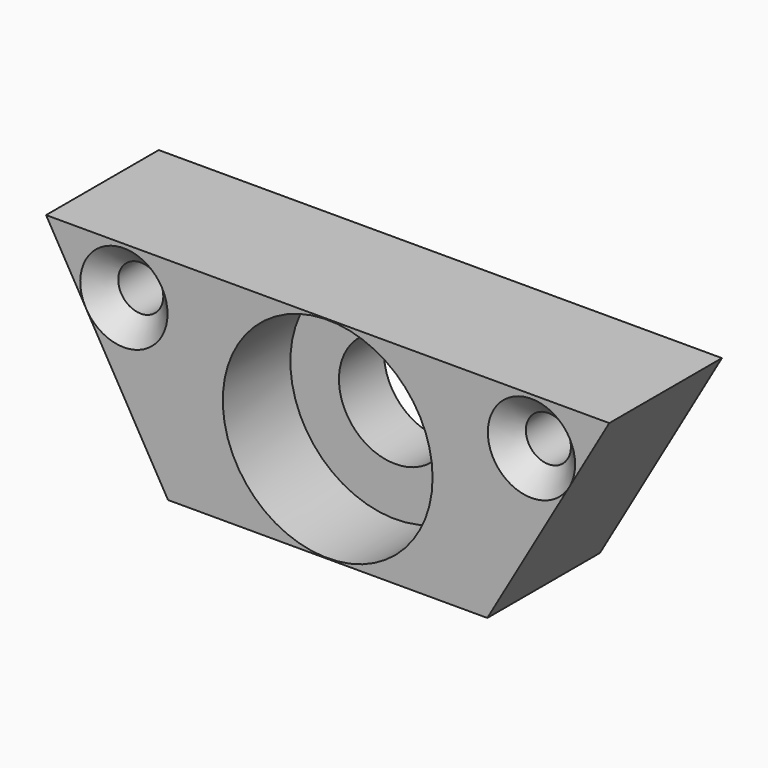
from build123d import *

# Parameters (mm, degrees)
F0_R     = 1.6
F0_R_2   = 4
F1_DEPTH = 10
F2_R     = 7.45
F2_R_2   = 4
F3_DEPTH = 6


# Not quite as in the source:
# - a fillet or chamfer that OpenCascade refuses, or shapes differently, is made with other operations: its cross-section is extruded or revolved along the edge and cut away or added


with BuildPart() as f1:
    # F0 (on Front) → F1 (new body)
    with BuildSketch(Plane.XZ):
        Polygon((20, 7.5), (-20, 7.5), (-11.3397459622, -7.5), (11.3397459622, -7.5), align=None)
        with Locations((-14.4742550328, 4.1231745854)):
            Circle(F0_R, mode=Mode.SUBTRACT)
        Circle(F0_R_2, mode=Mode.SUBTRACT)
        with Locations((14.4742550328, 4.1231745854)):
            Circle(F0_R, mode=Mode.SUBTRACT)
    extrude(amount=F1_DEPTH)

    # F2 (on face) → F3 (cut)
    with BuildSketch(Plane.XZ.offset(10)):
        Circle(F2_R)
        Circle(F2_R_2, mode=Mode.SUBTRACT)
    extrude(amount=-F3_DEPTH, mode=Mode.SUBTRACT)

    # F4: chamfer of 1.5 on 2 edges, made by hand

    # F4_s1 → F4_t2 (revolve, cut)
    with BuildSketch(Plane.XY.offset(4.1231745854)):
        Polygon((-11.3742550328, -10), (-12.8742550328, -8.5), (-12.8742550328, -10), align=None)
    revolve(axis=Axis((-14.4742550328, -10, 4.1231745854), (0, -1, 0)), mode=Mode.SUBTRACT)

    # F4_s3 → F4_t4 (revolve, cut)
    with BuildSketch(Plane.XY.offset(4.1231745854)):
        Polygon((17.5742550328, -10), (16.0742550328, -8.5), (16.0742550328, -10), align=None)
    revolve(axis=Axis((14.4742550328, -10, 4.1231745854), (0, -1, 0)), mode=Mode.SUBTRACT)


solid = f1.part
